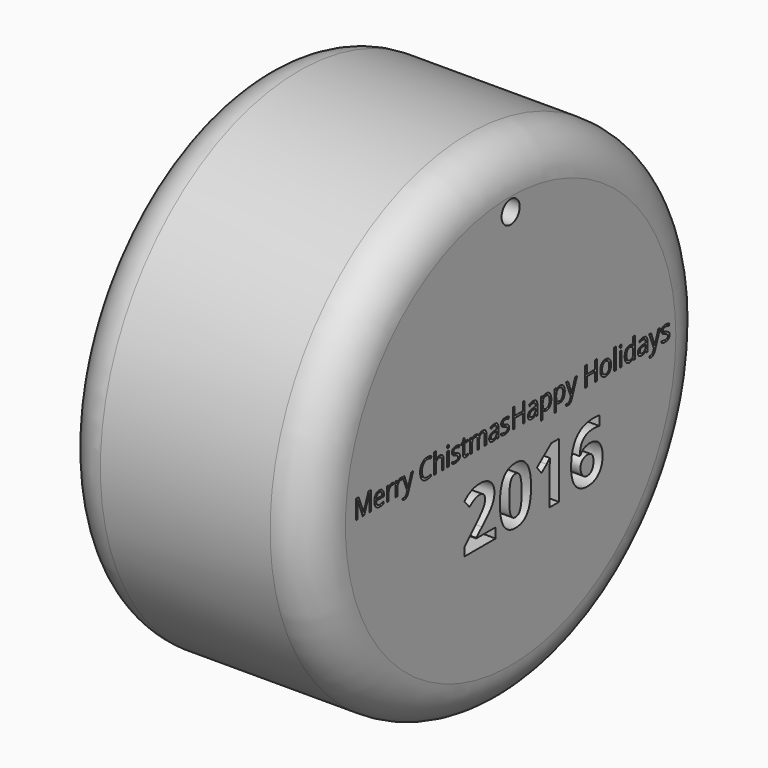
from build123d import *

# Parameters (mm, degrees)
F0_R           = 29.1284718783
F1_DEPTH       = 29.718
F2_R           = 4.9056819587
F4_TEXT_SIZE   = 3.1240048378
F4_TEXT_SIZE_2 = 3.2235056602
F4_TEXT_SIZE_3 = 9.1540982895
F5_DEPTH       = 5.334
F6_R           = 1.3256448848
F7_DEPTH       = 29.719
F8_DEPTH       = 1.6002
F9_TEXT_SIZE   = 6.0507781907
F10_TEXT_SIZE  = 6.0306572204
F11_DEPTH      = 25.4


# Not quite as in the source:
# - Text() gives the source's letters only with a copy of the font that has no kerning and outlines rounded to 1/6400 em; it was checked with that copy


with BuildPart() as f1:
    # F0 (on Right) → F1 (new body)
    with BuildSketch(Plane.YZ):
        Circle(F0_R)
    extrude(amount=-F1_DEPTH)

    # F2
    f2_edges = [f1.edges().sort_by_distance(p)[0] for p in [
        (0, -29.128472, 0),
        (-14.859, 29.128472, 0),
        (-29.718, -29.128472, 0),
    ]]
    fillet(f2_edges, radius=F2_R)

    # F4 (on face) → F5 (cut)
    with BuildSketch(Plane.YZ):
        with Locations((-22.9741268279, 0)):
            Text('Merry Chistmas', F4_TEXT_SIZE, font='Open Sans', text_align=(TextAlign.LEFT, TextAlign.BOTTOM))
        with Locations((0, 0)):
            Text('Happy Holidays', F4_TEXT_SIZE_2, font='Open Sans', text_align=(TextAlign.LEFT, TextAlign.BOTTOM))
        with Locations((-7.1293464862, -10.2162109688)):
            Text('2016', F4_TEXT_SIZE_3, font='Open Sans', font_style=FontStyle.BOLD, text_align=(TextAlign.LEFT, TextAlign.BOTTOM))
    extrude(amount=-F5_DEPTH, mode=Mode.SUBTRACT)

    # F6 (on face) → F7 (cut, through all)
    with BuildSketch(Plane.YZ):
        with Locations((0, 22.6194635034)):
            Circle(F6_R)
    extrude(amount=-F7_DEPTH, mode=Mode.SUBTRACT)

    # F3 (on face) → F8 (join)
    with BuildSketch(Plane(origin=(-29.718, 0, 0), x_dir=(0, -1, 0), z_dir=(-1, 0, 0))):
        Polygon((-3.9565147127, 0), (4.7093843153, 0), (0, 18.3828379959), align=None)
        Polygon((-13.4327909036, 0), (-5.5262172626, -7.293183464), (-3.9565147127, 0), align=None)
        Polygon((0.8322082884, -13.1583238132), (6.6316442138, -7.5034420499), (4.7093843153, 0), (-3.9565147127, 0), (-5.5262172626, -7.293183464), align=None)
        Polygon((-8.812678738, -22.5628066727), (0.8322082884, -13.1583238132), (-5.5262172626, -7.293183464), align=None)
        Polygon((0.8322082884, -13.1583238132), (10.3231220093, -21.9129346156), (6.6316442138, -7.5034420499), align=None)
        Polygon((4.7093843153, 0), (6.6316442138, -7.5034420499), (14.3268946558, 0), align=None)
    extrude(amount=F8_DEPTH)

    # F9 (on face) + F10 (on face) → F11 (cut)
    with BuildSketch(Plane(origin=(-29.718, 0, 0), x_dir=(0, -1, 0), z_dir=(-1, 0, 0))):
        with Locations((-16.0060413182, 3.5143047571)):
            Text('20', F9_TEXT_SIZE, font='Open Sans', font_style=FontStyle.BOLD, text_align=(TextAlign.LEFT, TextAlign.BOTTOM))
    with BuildSketch(Plane(origin=(-29.718, 0, 0), x_dir=(0, -1, 0), z_dir=(-1, 0, 0))):
        with Locations((7.291804222, 3.5215484228)):
            Text('16', F10_TEXT_SIZE, font='Open Sans', font_style=FontStyle.BOLD, text_align=(TextAlign.LEFT, TextAlign.BOTTOM))
    extrude(amount=-F11_DEPTH, mode=Mode.SUBTRACT)


solid = f1.part
